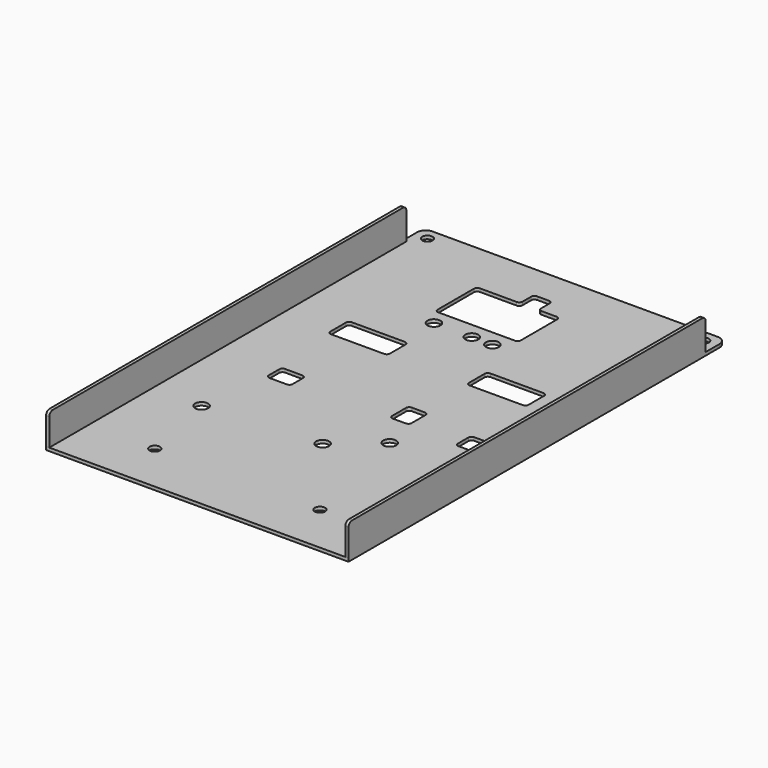
from build123d import *

# Parameters (mm, degrees)
F0_R     = 1.2
F0_R_2   = 1.5
F1_DEPTH = 0.744
F2_W     = 0.744
F2_H     = 103
F2_H_2   = 102.999995
F3_DEPTH = 8
F4_R     = 1


# Not quite as in the source:
# - ends of sketch curves that miss each other by under 0.0002 mm in the source are joined


with BuildPart() as f1:
    # F0 (on Top) → F1 (new body)
    with BuildSketch(Plane.XY):
        with BuildLine():
            Line((-39.500012, -54.499996), (30.29995, -54.500001))
            Line((30.29995, -54.500001), (30.29995, 52.4999855731))
            ThreePointArc((30.29995, 52.4999855731), (29.714163765, 53.9141989328), (28.2999505731, 54.4999855731))
            Line((28.2999505731, 54.4999855731), (-37.5000114269, 54.5000044269))
            ThreePointArc((-37.5000114269, 54.5000044269), (-38.9142253598, 53.9142181919), (-39.500012, 52.5000044269))
            Line((-39.500012, 52.5000044269), (-39.500012, -54.499996))
        make_face()
        with Locations((-23.649861, -42.950105)):
            Circle(F0_R, mode=Mode.SUBTRACT)
        with Locations((-27.501189, -24.642994)):
            Circle(F0_R_2, mode=Mode.SUBTRACT)
        with BuildLine():
            Line((-20.749991, -8.499996), (-24.749991, -8.499996))
            ThreePointArc((-24.749991, -8.499996), (-25.2803207323, -8.2803268537), (-25.499992, -7.749998))
            Line((-25.499992, -7.749998), (-25.499992, -4.749996))
            ThreePointArc((-25.499992, -4.749996), (-25.2803225001, -4.2196659141), (-24.749993, -3.999995))
            Line((-24.749993, -3.999995), (-20.749991, -3.999995))
            ThreePointArc((-20.749991, -3.999995), (-20.2196642677, -4.2196641463), (-19.999993, -4.749993))
            Line((-19.999993, -4.749993), (-19.999993, -7.749995))
            ThreePointArc((-19.999993, -7.749995), (-20.2196621463, -8.2803247323), (-20.749991, -8.499996))
        make_face(mode=Mode.SUBTRACT)
        with Locations((14.450063, -42.950105)):
            Circle(F0_R, mode=Mode.SUBTRACT)
        with Locations((-1.248788, -22.556994)):
            Circle(F0_R_2, mode=Mode.SUBTRACT)
        with Locations((8.00001, -14.749994)):
            Circle(F0_R_2, mode=Mode.SUBTRACT)
        with BuildLine():
            ThreePointArc((2.500013, -6.999991), (1.9696832677, -6.7803218537), (1.750012, -6.249993))
            Line((1.750012, -6.249993), (1.750012, -2.249993))
            ThreePointArc((1.750012, -2.249993), (1.9696814999, -1.7196629141), (2.500011, -1.499992))
            Line((2.500011, -1.499992), (5.500012, -1.499992))
            ThreePointArc((5.500012, -1.499992), (6.0303420859, -1.7196614999), (6.250013, -2.249991))
            Line((6.250013, -2.249991), (6.250013, -6.249993))
            ThreePointArc((6.250013, -6.249993), (6.0303438537, -6.7803197323), (5.500015, -6.999991))
            Line((5.500015, -6.999991), (2.500013, -6.999991))
        make_face(mode=Mode.SUBTRACT)
        with BuildLine():
            ThreePointArc((17.750011, -4.249994), (17.9696801463, -3.7196642677), (18.500009, -3.499993))
            Line((18.500009, -3.499993), (22.500011, -3.499993))
            ThreePointArc((22.500011, -3.499993), (23.0303390859, -3.7196624999), (23.25001, -4.249992))
            Line((23.25001, -4.249992), (23.25001, -7.249993))
            ThreePointArc((23.25001, -7.249993), (23.0303405001, -7.7803230859), (22.500011, -7.999994))
            Line((22.500011, -7.999994), (18.500012, -7.999995))
            ThreePointArc((18.500012, -7.999995), (17.9696822677, -7.7803248537), (17.750011, -7.249996))
            Line((17.750011, -7.249996), (17.750011, -4.249994))
        make_face(mode=Mode.SUBTRACT)
        with BuildLine():
            Line((-13.749987, 17.000004), (-13.749987, 12.500005))
            ThreePointArc((-13.749987, 12.500005), (-13.9696564999, 11.9696749141), (-14.499986, 11.750004))
            Line((-14.499986, 11.750004), (-26.749989, 11.750004))
            ThreePointArc((-26.749989, 11.750004), (-27.2803170859, 11.9696734999), (-27.499988, 12.500003))
            Line((-27.499988, 12.500003), (-27.499988, 17.000004))
            ThreePointArc((-27.499988, 17.000004), (-27.2803185001, 17.5303340859), (-26.749989, 17.750005))
            Line((-26.749989, 17.750005), (-14.499988, 17.750005))
            ThreePointArc((-14.499988, 17.750005), (-13.9696579141, 17.5303355001), (-13.749987, 17.000004))
        make_face(mode=Mode.SUBTRACT)
        with Locations((-14.999987, 26.750007)):
            Circle(F0_R_2, mode=Mode.SUBTRACT)
        with Locations((-6.249987, 26.750005)):
            Circle(F0_R_2, mode=Mode.SUBTRACT)
        with Locations((-36.499988, 51.750005)):
            Circle(F0_R, mode=Mode.SUBTRACT)
        with BuildLine():
            ThreePointArc((-16.999976, 30.499992), (-17.5303057323, 30.7196611463), (-17.749977, 31.24999))
            Line((-17.749977, 31.24999), (-17.749987, 41.749995))
            ThreePointArc((-17.749987, 41.749995), (-17.5303305001, 42.2803250859), (-17.000001, 42.499996))
            Line((-17.000001, 42.499996), (-8.499988, 42.500006))
            ThreePointArc((-8.499988, 42.500006), (-7.9696584999, 42.7196769141), (-7.749989, 43.250007))
            Line((-7.749989, 43.250007), (-7.749989, 45.750005))
            ThreePointArc((-7.749989, 45.750005), (-7.5303175001, 46.2803350859), (-6.999988, 46.500006))
            Line((-6.999988, 46.500006), (-4.249989, 46.500006))
            ThreePointArc((-4.249989, 46.500006), (-3.7196594999, 46.2803350859), (-3.49999, 45.750005))
            Line((-3.49999, 45.750005), (-3.499987, 43.250007))
            ThreePointArc((-3.499987, 43.250007), (-3.2803178537, 42.7196772677), (-2.749989, 42.500006))
            Line((-2.749989, 42.500006), (0.699984, 42.500006))
            ThreePointArc((0.699984, 42.500006), (1.2303137323, 42.2803368537), (1.449985, 41.750008))
            Line((1.449985, 41.750008), (1.449985, 41.250006))
            Line((1.449985, 41.250006), (1.449985, 31.24999))
            ThreePointArc((1.449985, 31.24999), (1.2303037323, 30.7196611463), (0.699974, 30.499992))
            Line((0.699974, 30.499992), (-16.999976, 30.499992))
        make_face(mode=Mode.SUBTRACT)
        with Locations((-1.499989, 26.750005)):
            Circle(F0_R_2, mode=Mode.SUBTRACT)
        with BuildLine():
            ThreePointArc((5.250013, 11.750004), (4.7196829141, 11.9696734999), (4.500012, 12.500003))
            Line((4.500012, 12.500003), (4.500012, 17.000004))
            ThreePointArc((4.500012, 17.000004), (4.7196811463, 17.5303337323), (5.25001, 17.750005))
            Line((5.25001, 17.750005), (17.500011, 17.750005))
            ThreePointArc((17.500011, 17.750005), (18.0303410859, 17.5303355001), (18.250012, 17.000006))
            Line((18.250012, 17.000006), (18.250012, 12.500005))
            ThreePointArc((18.250012, 12.500005), (18.0303428537, 11.9696752677), (17.500014, 11.750004))
            Line((17.500014, 11.750004), (5.250013, 11.750004))
        make_face(mode=Mode.SUBTRACT)
        with Locations((27.250012, 51.750005)):
            Circle(F0_R, mode=Mode.SUBTRACT)
    extrude(amount=F1_DEPTH)

    # F2 (on face) → F3 (join)
    with BuildSketch(Plane(origin=(0, 0, 0), x_dir=(1, 0, 0), z_dir=(0, 0, -1))):
        with Locations((29.92795, 3.000001)):
            Rectangle(F2_W, F2_H)
        with Locations((-39.128012, 2.9999985)):
            Rectangle(F2_W, F2_H_2)
    extrude(amount=-F3_DEPTH)

    # F4
    f4_edges = [f1.edges().sort_by_distance(p)[0] for p in [
        (29.92795, -54.500001, 8),
        (29.92795, 48.499999, 8),
        (-39.128012, 48.499999, 8),
        (-39.128012, -54.499996, 8),
    ]]
    fillet(f4_edges, radius=F4_R)


solid = f1.part
